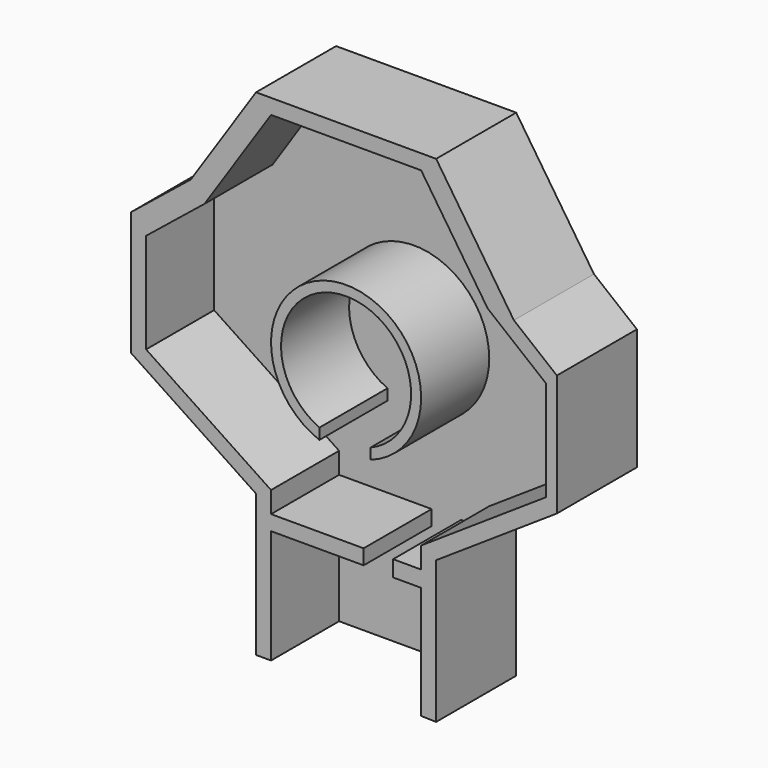
from build123d import *

# Parameters (mm, degrees)
F1_DEPTH  = 25.4
F2_DEPTH  = 25.4
F3_DEPTH  = 3.81
F5_W      = 23.4985564016
F5_H      = 3.8088811561
F5_W_2    = 7.119712124
F5_H_2    = 4.0809446946
F6_DEPTH  = 21.59
F7_W      = 1.7024531355
F7_H      = 9.2860683799
F8_DEPTH  = 2.54
F9_W      = 2.2018989548
F9_H      = 9.2860683799
F10_DEPTH = 3.175
F11_DEPTH = 3.175
F12_W     = 2.2159516811
F12_H     = 9.2260986567
F12_W_2   = 2.2018989548
F13_DEPTH = 3.175
F14_W     = 2.208925318
F14_H     = 9.2260986567
F14_W_2   = 2.2090896964
F15_DEPTH = 3.175
F16_W     = 2.1525025368
F16_H     = 9.2260986567
F16_W_2   = 2.2090075072
F17_DEPTH = 3.175
F18_W     = 2.180755022
F18_H     = 9.2260986567
F18_W_2   = 2.1889545023
F19_DEPTH = 3.175
F20_W     = 2.1348558366
F20_H     = 9.2260986567
F20_W_2   = 2.1848547622
F21_DEPTH = 3.175
F22_W     = 2.1598552994
F22_H     = 9.1612674296
F22_W_2   = 2.1560452878
F23_DEPTH = 3.175
F24_DEPTH = 3.81


with BuildPart() as f1:
    # F0 (on Front) → F1 (new body)
    with BuildSketch(Plane.XZ):
        Polygon((-71.3886133739, 62.7737028413), (-67.9131094975, 58.461044946), (-51.0271422677, 83.8361215117), (-54.8371422677, 87.6461215117), align=None)
        Polygon((-86.5559879748, 50.5505517126), (-82.7459879748, 46.5074590373), (-67.9131094975, 58.461044946), (-71.3886133739, 62.7737028413), align=None)
        Polygon((-86.5559879748, 19.0663513101), (-82.7459879748, 21.1074590373), (-82.7459879748, 46.5074590373), (-86.5559879748, 50.5505517126), align=None)
        Polygon((-54.8371422677, -2.0411077271), (-51.0271422677, 0), (-82.7459879748, 21.1074590373), (-86.5559879748, 19.0663513101), align=None)
        Polygon((-51.0271422677, -9.4391499932), (-51.0271422677, 0), (-54.8371422677, -2.0411077271), (-54.8371422677, -38.1), (-51.0271422677, -38.1), align=None)
        Polygon((-54.8371422677, 87.6461215117), (-51.0271422677, 83.8361215117), (-12.9271422677, 83.8361215117), (-9.1171422677, 87.6461215117), align=None)
        Polygon((-9.1171422677, 87.6461215117), (-12.9271422677, 83.8361215117), (3.9588249621, 58.461044946), (10.6205295243, 57.9856983845), align=None)
        Polygon((10.6205295243, 57.9856983845), (3.9588249621, 58.461044946), (18.7917034394, 46.5074590373), (21.5305625329, 49.1934725845), align=None)
        Polygon((18.7917034394, 46.5074590373), (18.7917034394, 21.1074590373), (21.5305625329, 18.3535554217), (21.5305625329, 49.1934725845), align=None)
        Polygon((18.7917034394, 21.1074590373), (-12.9271422677, 0), (-9.1171422677, -2.0411077271), (21.5305625329, 18.3535554217), align=None)
        Polygon((-12.9271422677, -9.4391499932), (-12.9271422677, -38.1), (-9.1171422677, -38.1877794862), (-9.1171422677, -2.0411077271), (-12.9271422677, 0), align=None)
    extrude(amount=F1_DEPTH)

    # F0 (on Front) → F3 (join)
    with BuildSketch(Plane.XZ):
        Polygon((-82.7459879748, 21.1074590373), (-51.0271422677, 0), (-51.0271422677, -9.4391499932), (-51.0271422677, -38.1), (-12.9271422677, -38.1), (-12.9271422677, -9.4391499932), (-12.9271422677, 0), (18.7917034394, 21.1074590373), (18.7917034394, 46.5074590373), (3.9588249621, 58.461044946), (-12.9271422677, 83.8361215117), (-51.0271422677, 83.8361215117), (-67.9131094975, 58.461044946), (-82.7459879748, 46.5074590373), align=None)
        with BuildLine():
            ThreePointArc((-38.7432127325, 15.1876261035), (-31.6836311373, 52.0835575626), (-25.7617975071, 14.988014205))
            Line((-25.7617975071, 14.988014205), (-25.7617975071, 17.7207682707))
            ThreePointArc((-25.7617975071, 17.7207682707), (-31.676990567, 49.5235857889), (-38.7432127325, 17.9565584449))
            Line((-38.7432127325, 17.9565584449), (-38.7432127325, 15.1876261035))
        make_face(mode=Mode.SUBTRACT)
        Polygon((-23.7218233431, 32.9955678842), (-31.9771422677, 32.9955678842), (-40.2319762915, 32.9955678842), (-40.2319762915, 42.3252284527), (-23.7218233431, 42.3252284527), (-23.7218233431, 33.0163085965), align=None, mode=Mode.SUBTRACT)
    extrude(amount=F3_DEPTH)

    # F5 (on face) → F6 (join)
    with BuildSketch(Plane.XZ.offset(3.81)):
        with Locations((-39.2778640669, -7.2833341546)):
            Rectangle(F5_W, F5_H)
        with Locations((-16.4869983297, -7.4193659239)):
            Rectangle(F5_W_2, F5_H_2)
    extrude(amount=F6_DEPTH)


with BuildPart() as f2:
    # F0 (on Front) → F2 (new body, symmetric)
    with BuildSketch(Plane.XZ):
        with BuildLine():
            Line((-25.7617975071, 17.7207682707), (-25.7617975071, 14.988014205))
            ThreePointArc((-25.7617975071, 14.988014205), (-31.6842499191, 52.043316152), (-38.7432127325, 15.1876261035))
            Line((-38.7432127325, 15.1876261035), (-38.7432127325, 17.9565584449))
            ThreePointArc((-38.7432127325, 17.9565584449), (-31.676990567, 49.5235857889), (-25.7617975071, 17.7207682707))
        make_face()
    extrude(amount=F2_DEPTH, both=True)

    # F4 (on face) → F24, piece 2 (join)
    with BuildSketch(Plane(origin=(0, 25.4, 0), x_dir=(-1, 0, 0), z_dir=(0, 1, 0))):
        with BuildLine():
            ThreePointArc((25.7617975071, 16.8035637745), (22.1389603555, 47.3235128183), (49.3399924318, 33.0163085965))
            ThreePointArc((49.3399924318, 33.0163085965), (46.4503440601, 23.4248103372), (38.7432127325, 17.0258234433))
            Line((38.7432127325, 17.0258234433), (38.7432127325, 15.1876261035))
            ThreePointArc((38.7432127325, 15.1876261035), (31.6842499191, 52.043316152), (25.7617975071, 14.988014205))
            Line((25.7617975071, 14.988014205), (25.7617975071, 16.8035637745))
        make_face()
    extrude(amount=F24_DEPTH)


with BuildPart() as f8:
    # F7 (on face) → F8 (new body, symmetric)
    with BuildSketch(Plane.XZ):
        with Locations((-24.5730499108, 37.6821942627)):
            Rectangle(F7_W, F7_H)
    extrude(amount=F8_DEPTH, both=True)

    # F9 (on face) → F10 (join)
    with BuildSketch(Plane(origin=(0, 2.54, 0), x_dir=(-1, 0, 0), z_dir=(0, 1, 0))):
        with Locations((26.525225956, 37.6821942627)):
            Rectangle(F9_W, F9_H)
    extrude(amount=F10_DEPTH)

    # F11 (add): a face of the model
    f11_faces = [f8.faces().sort_by_distance(p)[0] for p in [
        (-24.5730499108, 2.54, 37.6821942627),
    ]]
    extrude(f11_faces, amount=F11_DEPTH)

    # F12 (on face) → F13 (join)
    with BuildSketch(Plane(origin=(0, 5.715, 0), x_dir=(-1, 0, 0), z_dir=(0, 1, 0))):
        with Locations((28.734151274, 37.7121791244)):
            Rectangle(F12_W, F12_H)
        with Locations((26.525225956, 37.7121791244)):
            Rectangle(F12_W_2, F12_H)
    extrude(amount=F13_DEPTH)

    # F14 (on face) → F15 (join)
    with BuildSketch(Plane(origin=(0, 8.89, 0), x_dir=(-1, 0, 0), z_dir=(0, 1, 0))):
        with Locations((28.7376644555, 37.7121791244)):
            Rectangle(F14_W, F14_H)
        with Locations((30.9466719627, 37.7121791244)):
            Rectangle(F14_W_2, F14_H)
    extrude(amount=F15_DEPTH)

    # F16 (on face) → F17 (join)
    with BuildSketch(Plane(origin=(0, 12.065, 0), x_dir=(-1, 0, 0), z_dir=(0, 1, 0))):
        with Locations((33.1274680793, 37.7121791244)):
            Rectangle(F16_W, F16_H)
        with Locations((30.9467130573, 37.7121791244)):
            Rectangle(F16_W_2, F16_H)
    extrude(amount=F17_DEPTH)

    # F18 (on face) → F19 (join)
    with BuildSketch(Plane(origin=(0, 15.24, 0), x_dir=(-1, 0, 0), z_dir=(0, 1, 0))):
        with Locations((33.1133418367, 37.7121791244)):
            Rectangle(F18_W, F18_H)
        with Locations((35.2981965989, 37.7121791244)):
            Rectangle(F18_W_2, F18_H)
    extrude(amount=F19_DEPTH)

    # F20 (on face) → F21 (join)
    with BuildSketch(Plane(origin=(0, 18.415, 0), x_dir=(-1, 0, 0), z_dir=(0, 1, 0))):
        with Locations((37.4601017684, 37.7121791244)):
            Rectangle(F20_W, F20_H)
        with Locations((35.300246469, 37.7121791244)):
            Rectangle(F20_W_2, F20_H)
    extrude(amount=F21_DEPTH)

    # F22 (on face) → F23 (join)
    with BuildSketch(Plane(origin=(0, 21.59, 0), x_dir=(-1, 0, 0), z_dir=(0, 1, 0))):
        with Locations((37.447602037, 37.7445947379)):
            Rectangle(F22_W, F22_H)
        with Locations((39.6055523306, 37.7445947379)):
            Rectangle(F22_W_2, F22_H)
    extrude(amount=F23_DEPTH)


with BuildPart() as f24:
    # F4 (on face) → F24 (new body)
    with BuildSketch(Plane(origin=(0, 25.4, 0), x_dir=(-1, 0, 0), z_dir=(0, 1, 0))):
        with BuildLine():
            Line((25.7617975071, 17.7207682707), (25.7617975071, 16.8035637745))
            ThreePointArc((25.7617975071, 16.8035637745), (32.2740610966, 15.6556838807), (38.7432127325, 17.0258234433))
            Line((38.7432127325, 17.0258234433), (38.7432127325, 17.9565584449))
            ThreePointArc((38.7432127325, 17.9565584449), (31.676990567, 49.5235857889), (25.7617975071, 17.7207682707))
        make_face()
    extrude(amount=F24_DEPTH)


solid = Compound([f1.part, f2.part, f8.part, f24.part])
